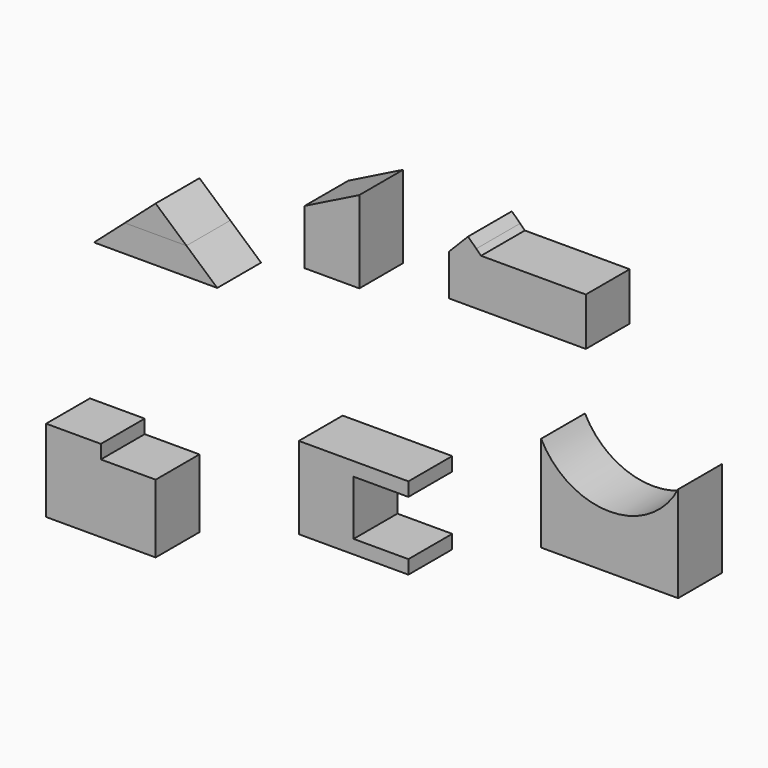
from build123d import *

# Parameters (mm, degrees)
F2_DEPTH  = 101.6
F4_DEPTH  = 101.6
F6_DEPTH  = 101.6
F8_DEPTH  = 101.6
F10_DEPTH = 101.6


with BuildPart() as f2:
    # F0 (on Front) → F2 (new body)
    with BuildSketch(Plane.XZ):
        Polygon((57.15, -50.4015624758), (0, 0), (-57.15, -50.4015624758), align=None)
    extrude(amount=F2_DEPTH)


with BuildPart() as f2b:
    # F1 (on face) → F2, piece 2 (new body)
    with BuildSketch(Plane.XZ):
        Polygon((114.3, -100.8031249516), (57.15, -50.4015624758), (-57.15, -50.4015624758), (-114.3, -100.8031249516), align=None)
    extrude(amount=F2_DEPTH)


with BuildPart() as f4:
    # F3 (on Front) → F4 (new body)
    with BuildSketch(Plane.XZ):
        Polygon((377.7606872082, -15.8657720208), (377.7606872082, 136.5342279792), (276.1606872082, 85.7342279792), (276.1606872082, -15.8657720208), align=None)
    extrude(amount=F4_DEPTH)


with BuildPart() as f4b:
    # F3 (on Front) → F4, piece 2 (new body)
    with BuildSketch(Plane.XZ):
        Polygon((543.8886880875, 98.1160318375), (543.8886880875, 21.9160318375), (594.6886880875, 21.9160318375), (594.6886880875, 72.7160318375), (594.6886880875, 119.4656812943), (579.4372981796, 134.4056490925), align=None)
        Polygon((603.5186386078, 110.8160318375), (642.4128292338, 72.7160318375), (797.8886880875, 72.7160318375), (797.8886880875, 110.8160318375), align=None)
        Polygon((594.6886880875, 72.7160318375), (594.6886880875, 21.9160318375), (645.4886880875, 21.9160318375), (797.8886880875, 21.9160318375), (797.8886880875, 72.7160318375), (642.4128292338, 72.7160318375), align=None)
        Polygon((594.6886880875, 119.4656812943), (594.6886880875, 72.7160318375), (642.4128292338, 72.7160318375), (603.5186386078, 110.8160318375), align=None)
    extrude(amount=F4_DEPTH)


with BuildPart() as f6:
    # F5 (on Front) → F6 (new body)
    with BuildSketch(Plane.XZ):
        Polygon((-101.6, -425.6145358086), (-203.2, -425.6145358086), (-203.2, -578.0145358086), (0, -578.0145358086), (0, -451.0145358086), (-101.6, -451.0145358086), align=None)
    extrude(amount=F6_DEPTH)


with BuildPart() as f8:
    # F7 (on Front) → F8 (new body)
    with BuildSketch(Plane.XZ):
        Polygon((468.7846178532, -301.2978369474), (265.5846178532, -301.2978369474), (265.5846178532, -453.6978369474), (468.7846178532, -453.6978369474), (468.7846178532, -428.2978369474), (367.1846178532, -428.2978369474), (367.1846178532, -326.6978369474), (468.7846178532, -326.6978369474), align=None)
    extrude(amount=F8_DEPTH)


with BuildPart() as f10:
    # F9 (on Front) → F10 (new body)
    with BuildSketch(Plane.XZ):
        with BuildLine():
            ThreePointArc((968.9937152863, -151.64017663), (841.9937152863, -229.2261491845), (714.9937152863, -151.64017663))
            Line((714.9937152863, -151.64017663), (714.9937152863, -329.44017663))
            Line((714.9937152863, -329.44017663), (968.9937152863, -329.44017663))
            Line((968.9937152863, -329.44017663), (968.9937152863, -151.64017663))
        make_face()
    extrude(amount=F10_DEPTH)


solid = Compound([f2.part, f2b.part, f4.part, f4b.part, f6.part, f8.part, f10.part])
